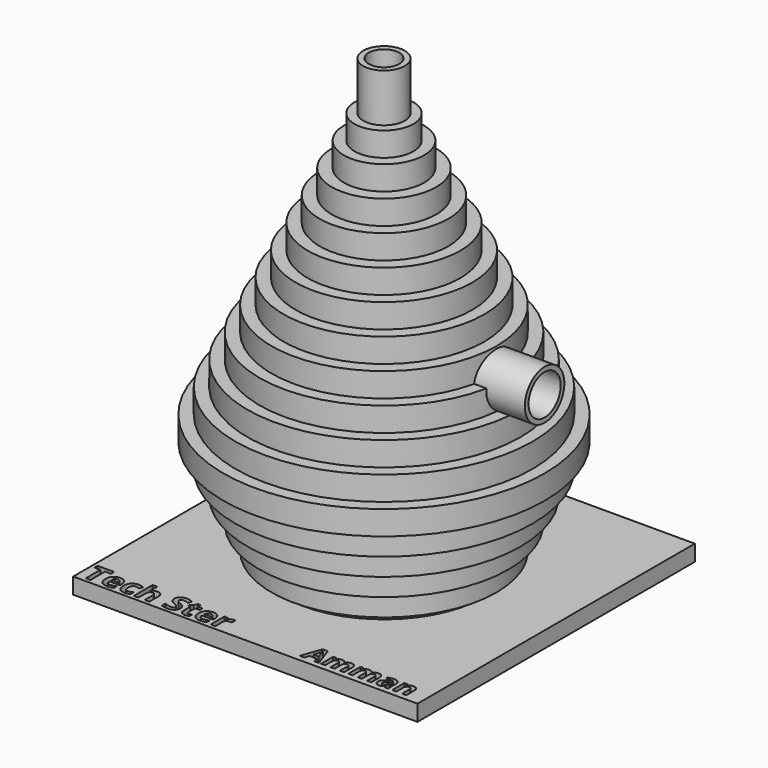
from build123d import *

# Parameters (mm, degrees)
F0_R          = 12.5
F1_DEPTH      = 3
F2_R          = 14
F3_DEPTH      = 3
F4_R          = 15.5
F5_DEPTH      = 3
F6_R          = 17
F7_DEPTH      = 3
F8_R          = 18.5
F9_DEPTH      = 3
F10_R         = 20
F11_DEPTH     = 3
F12_R         = 18.5
F13_DEPTH     = 3
F14_R         = 17
F15_DEPTH     = 3
F16_R         = 15.5
F17_DEPTH     = 3
F18_R         = 14
F19_DEPTH     = 3
F20_R         = 12.5
F21_DEPTH     = 3
F22_R         = 11
F23_DEPTH     = 3
F24_R         = 9.5
F25_DEPTH     = 3
F26_R         = 8
F27_DEPTH     = 3
F28_R         = 6.5
F29_DEPTH     = 3
F31_W         = 42.8677387536
F31_H         = 43.161354959
F32_DEPTH     = 2
F33_TEXT_SIZE = 3.8513887881
F34_DEPTH     = 25.4
F35_TEXT_SIZE = 3.4521049302
F36_DEPTH     = 25.4
F30_R         = 5
F37_DEPTH     = 3
F38_R         = 3.6702439253
F39_DEPTH     = 3
F40_R         = 2.5831943807
F41_DEPTH     = 6
F42_R         = 1.9006943823
F43_DEPTH     = 52.324
F44_R         = 3.072461612
F45_DEPTH     = 20
F46_R         = 2.49824525
F47_DEPTH     = 25.4


# Not quite as in the source:
# - Text() gives the source's letters only with a copy of the font that has no kerning and outlines rounded to 1/6400 em; it was checked with that copy


with BuildPart() as f1:
    # F0 (on Top) → F1 (new body)
    with BuildSketch(Plane.XY):
        Circle(F0_R)
    extrude(amount=F1_DEPTH)

    # F2 (on face) → F3 (join)
    with BuildSketch(Plane.XY.offset(3)):
        Circle(F2_R)
    extrude(amount=F3_DEPTH)

    # F4 (on face) → F5 (join)
    with BuildSketch(Plane.XY.offset(6)):
        Circle(F4_R)
    extrude(amount=F5_DEPTH)

    # F6 (on face) → F7 (join)
    with BuildSketch(Plane.XY.offset(9)):
        Circle(F6_R)
    extrude(amount=F7_DEPTH)

    # F8 (on face) → F9 (join)
    with BuildSketch(Plane.XY.offset(12)):
        Circle(F8_R)
    extrude(amount=F9_DEPTH)

    # F10 (on face) → F11 (join)
    with BuildSketch(Plane.XY.offset(15)):
        Circle(F10_R)
    extrude(amount=F11_DEPTH)

    # F12 (on face) → F13 (join)
    with BuildSketch(Plane.XY.offset(18)):
        Circle(F12_R)
    extrude(amount=F13_DEPTH)

    # F14 (on face) → F15 (join)
    with BuildSketch(Plane.XY.offset(21)):
        Circle(F14_R)
    extrude(amount=F15_DEPTH)

    # F16 (on face) → F17 (join)
    with BuildSketch(Plane.XY.offset(24)):
        Circle(F16_R)
    extrude(amount=F17_DEPTH)

    # F18 (on face) → F19 (join)
    with BuildSketch(Plane.XY.offset(27)):
        Circle(F18_R)
    extrude(amount=F19_DEPTH)

    # F20 (on face) → F21 (join)
    with BuildSketch(Plane.XY.offset(30)):
        Circle(F20_R)
    extrude(amount=F21_DEPTH)

    # F22 (on face) → F23 (join)
    with BuildSketch(Plane.XY.offset(33)):
        Circle(F22_R)
    extrude(amount=F23_DEPTH)

    # F24 (on face) → F25 (join)
    with BuildSketch(Plane.XY.offset(36)):
        Circle(F24_R)
    extrude(amount=F25_DEPTH)

    # F26 (on face) → F27 (join)
    with BuildSketch(Plane.XY.offset(39)):
        Circle(F26_R)
    extrude(amount=F27_DEPTH)

    # F28 (on face) → F29 (join)
    with BuildSketch(Plane.XY.offset(42)):
        Circle(F28_R)
    extrude(amount=F29_DEPTH)

    # F31 (on face) → F32 (join)
    with BuildSketch(Plane(origin=(0, 0, 0), x_dir=(1, 0, 0), z_dir=(0, 0, -1))):
        Rectangle(F31_W, F31_H)
    extrude(amount=-F32_DEPTH)

    # F33 (on face) → F34 (cut)
    with BuildSketch(Plane.XY.offset(2)):
        with Locations((-21.0731877014, -21.0926905274)):
            Text('Tech Ster', F33_TEXT_SIZE, font='Open Sans', font_style=FontStyle.BOLD, text_align=(TextAlign.LEFT, TextAlign.BOTTOM))
    extrude(amount=-F34_DEPTH, mode=Mode.SUBTRACT)

    # F35 (on face) → F36 (cut)
    with BuildSketch(Plane.XY.offset(2)):
        with Locations((6.209728308, -20.8713710308)):
            Text('Amman', F35_TEXT_SIZE, font='Open Sans', font_style=FontStyle.BOLD, text_align=(TextAlign.LEFT, TextAlign.BOTTOM))
    extrude(amount=-F36_DEPTH, mode=Mode.SUBTRACT)

    # F30 (on face) → F37 (join)
    with BuildSketch(Plane.XY.offset(45)):
        Circle(F30_R)
    extrude(amount=F37_DEPTH)

    # F38 (on face) → F39 (join)
    with BuildSketch(Plane.XY.offset(48)):
        Circle(F38_R)
    extrude(amount=F39_DEPTH)

    # F40 (on face) → F41 (join)
    with BuildSketch(Plane.XY.offset(51)):
        Circle(F40_R)
    extrude(amount=F41_DEPTH)

    # F42 (on face) → F43 (cut)
    with BuildSketch(Plane.XY.offset(57)):
        Circle(F42_R)
    extrude(amount=-F43_DEPTH, mode=Mode.SUBTRACT)

    # F44 (on Right) → F45 (join)
    with BuildSketch(Plane.YZ):
        with Locations((0, 26.6248434782)):
            Circle(F44_R)
    extrude(amount=F45_DEPTH)

    # F46 (on face) → F47 (cut)
    with BuildSketch(Plane.YZ.offset(20)):
        with Locations((0, 26.6248434782)):
            Circle(F46_R)
    extrude(amount=-F47_DEPTH, mode=Mode.SUBTRACT)


solid = f1.part
